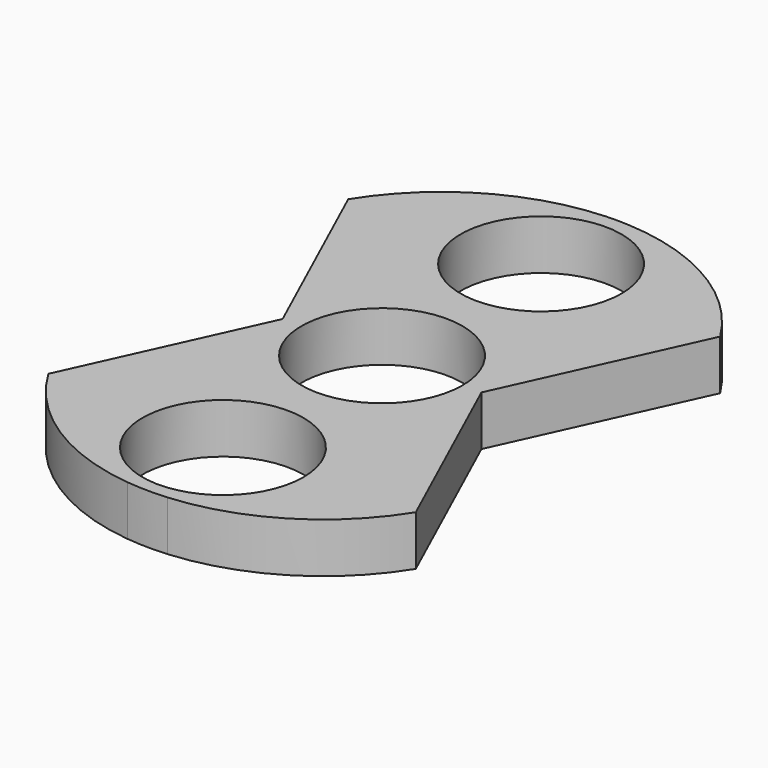
from build123d import *

# Parameters (mm, degrees)
F0_R     = 11.303
F1_DEPTH = 7.0104


# Not quite as in the source:
# - a feature names something its author has since deleted; it is built from what else it names


with BuildPart() as f1:
    # F0 (on Top) → F1 (new body)
    with BuildSketch(Plane.XY):
        with BuildLine():
            ThreePointArc((-8.4576062893, 17.6302414744), (0, 14.605), (8.4576062893, 17.6302414744))
            ThreePointArc((8.4576062893, 17.6302414744), (12.0541363205, 22.2373670497), (13.335, 27.94))
            ThreePointArc((13.335, 27.94), (9.9631286308, 36.8033116207), (1.552728851, 41.1842915294))
            ThreePointArc((1.552728851, 41.1842915294), (0, 41.2234534857), (-1.552728851, 41.1842915294))
            ThreePointArc((-1.552728851, 41.1842915294), (-12.7964847088, 31.6912936565), (-8.4576062893, 17.6302414744))
        make_face()
        with Locations((0, 27.94)):
            Circle(F0_R, mode=Mode.SUBTRACT)
        with BuildLine():
            ThreePointArc((-8.4410840797, 11.1314419353), (0, 13.97), (8.4410840797, 11.1314419353))
            ThreePointArc((8.4410840797, 11.1314419353), (7.023943937, 14.3844655708), (8.4576062893, 17.6302414744))
            ThreePointArc((8.4576062893, 17.6302414744), (0, 14.605), (-8.4576062893, 17.6302414744))
            ThreePointArc((-8.4576062893, 17.6302414744), (-7.1686601212, 14.3840976519), (-8.4410840797, 11.1314419353))
        make_face()
        with BuildLine():
            ThreePointArc((8.4410840797, -11.1314419353), (12.5116514616, -6.2144571527), (13.97, 0))
            ThreePointArc((13.97, 0), (12.5116514616, 6.2144571527), (8.4410840797, 11.1314419353))
            ThreePointArc((8.4410840797, 11.1314419353), (0, 13.97), (-8.4410840797, 11.1314419353))
            ThreePointArc((-8.4410840797, 11.1314419353), (-12.5116514616, 6.2144571527), (-13.97, 0))
            ThreePointArc((-13.97, 0), (-12.5116514616, -6.2144571527), (-8.4410840797, -11.1314419353))
            ThreePointArc((-8.4410840797, -11.1314419353), (0, -13.97), (8.4410840797, -11.1314419353))
        make_face()
        Circle(F0_R, mode=Mode.SUBTRACT)
        with BuildLine():
            ThreePointArc((8.4410840797, -17.616709606), (7.0831122532, -14.3740757706), (8.4410840797, -11.1314419353))
            ThreePointArc((8.4410840797, -11.1314419353), (0, -13.97), (-8.4410840797, -11.1314419353))
            ThreePointArc((-8.4410840797, -11.1314419353), (-7.1012049909, -14.3740757706), (-8.4410840797, -17.616709606))
            ThreePointArc((-8.4410840797, -17.616709606), (0, -14.605), (8.4410840797, -17.616709606))
        make_face()
        with BuildLine():
            ThreePointArc((13.335, -27.94), (12.0495659922, -22.2277163587), (8.4410840797, -17.616709606))
            ThreePointArc((8.4410840797, -17.616709606), (0, -14.605), (-8.4410840797, -17.616709606))
            ThreePointArc((-8.4410840797, -17.616709606), (-12.9933407259, -30.9392201953), (-3.0623665698, -40.9186030062))
            ThreePointArc((-3.0623665698, -40.9186030062), (-0.2065651455, -41.0979009929), (2.6534571531, -41.0083354004))
            ThreePointArc((2.6534571531, -41.0083354004), (10.3248747241, -36.3791461021), (13.335, -27.94))
        make_face()
        with Locations((0, -27.94)):
            Circle(F0_R, mode=Mode.SUBTRACT)
        with BuildLine():
            ThreePointArc((-13.97, 0), (-12.5116514616, 6.2144571527), (-8.4410840797, 11.1314419353))
            ThreePointArc((-8.4410840797, 11.1314419353), (-7.1686601212, 14.3840976519), (-8.4576062893, 17.6302414744))
            ThreePointArc((-8.4576062893, 17.6302414744), (-12.7964847088, 31.6912936565), (-1.552728851, 41.1842915294))
            ThreePointArc((-1.552728851, 41.1842915294), (-15.6144282797, 36.9723347017), (-26.1298660189, 26.7303846776))
            Line((-26.1298660189, 26.7303846776), (-13.97, 0))
        make_face()
        with BuildLine():
            ThreePointArc((8.4410840797, 11.1314419353), (12.5116514616, 6.2144571527), (13.97, 0))
            Line((13.97, 0), (26.1298660189, 26.7303846776))
            ThreePointArc((26.1298660189, 26.7303846776), (15.6144282797, 36.9723347017), (1.552728851, 41.1842915294))
            ThreePointArc((1.552728851, 41.1842915294), (9.9631286308, 36.8033116207), (13.335, 27.94))
            ThreePointArc((13.335, 27.94), (12.0541363205, 22.2373670497), (8.4576062893, 17.6302414744))
            ThreePointArc((8.4576062893, 17.6302414744), (7.023943937, 14.3844655708), (8.4410840797, 11.1314419353))
        make_face()
        with BuildLine():
            Line((26.1298660189, -26.7303846776), (13.97, 0))
            ThreePointArc((13.97, 0), (12.5116514616, -6.2144571527), (8.4410840797, -11.1314419353))
            ThreePointArc((8.4410840797, -11.1314419353), (7.0831122532, -14.3740757706), (8.4410840797, -17.616709606))
            ThreePointArc((8.4410840797, -17.616709606), (12.0495659922, -22.2277163587), (13.335, -27.94))
            ThreePointArc((13.335, -27.94), (10.3248747241, -36.3791461021), (2.6534571531, -41.0083354004))
            ThreePointArc((2.6534571531, -41.0083354004), (16.0937498742, -36.6680054018), (26.1298660189, -26.7303846776))
        make_face()
        with BuildLine():
            ThreePointArc((-8.4410840797, -17.616709606), (-7.1012049909, -14.3740757706), (-8.4410840797, -11.1314419353))
            ThreePointArc((-8.4410840797, -11.1314419353), (-12.5116514616, -6.2144571527), (-13.97, 0))
            Line((-13.97, 0), (-25.8976111474, -26.2198311856))
            ThreePointArc((-25.8976111474, -26.2198311856), (-16.209405425, -36.2559483923), (-3.0623665698, -40.9186030062))
            ThreePointArc((-3.0623665698, -40.9186030062), (-12.9933407259, -30.9392201953), (-8.4410840797, -17.616709606))
        make_face()
    extrude(amount=F1_DEPTH)


solid = f1.part
